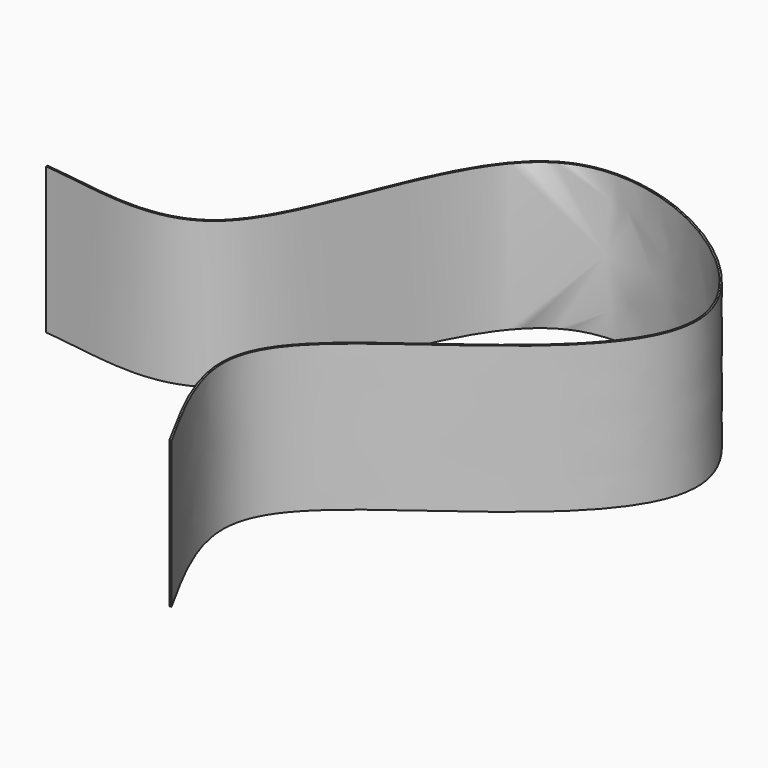
from build123d import *

# Parameters (mm, degrees)
F0_W     = 100
F0_H     = 70
F1_DEPTH = 16
F3_DEPTH = 25
F4_T     = -0.2
F5_DEPTH = 1


# Not quite as in the source:
# - a feature names something its author has since deleted; it is built from what else it names


with BuildPart() as f1:
    # F0 (on Top) → F1 (new body)
    with BuildSketch(Plane.XY):
        with Locations((0.9821429849, 33.5462264796)):
            Rectangle(F0_W, F0_H)
    extrude(amount=F1_DEPTH)

    # F2 (on face) → F3 (cut)
    with BuildSketch(Plane.XY.offset(16)):
        with BuildLine():
            Line((-49.0178570151, 68.5462264796), (-49.0178570151, 32.7192223562))
            add(Edge.make_bspline(
                [(-49.0178570151, 32.7192223562), (-43.4292364383, 32.2301652848), (-25.9811441186, 26.5813131518), (-21.7780426464, 74.7917895904), (26.8126262734, 45.2777093392), (-8.5734588785, 24.5947279779), (-17.4776549017, 13.6217093611), (-10.3822594237, 2.3846505635), (-8.3802593872, -1.4537735204)],
                knots=[0, 0, 0, 0, 0.1488243606, 0.3481063954, 0.5419458019, 0.7332399063, 0.8617053586, 1, 1, 1, 1], degree=3))
            Line((-8.3802593872, -1.4537735204), (50.9821429849, -1.4537735204))
            Line((50.9821429849, -1.4537735204), (50.9821429849, 68.5462264796))
            Line((50.9821429849, 68.5462264796), (-49.0178570151, 68.5462264796))
        make_face()
    extrude(amount=-F3_DEPTH, mode=Mode.SUBTRACT)

    # F4
    f4_openings = [f1.faces().sort_by_distance(p)[0] for p in [
        (-20.309609, 28.197223, 16),
        (-20.315883, 28.187702, 0),
        (-49.017857, 15.632724, 8),
    ]]
    offset(amount=F4_T, openings=f4_openings, kind=Kind.INTERSECTION)

    # F5 (cut): a face of the model
    f5_faces = [f1.faces().sort_by_distance(p)[0] for p in [
        (-28.6990582012, -1.4537735204, 8),
    ]]
    extrude(f5_faces, amount=-F5_DEPTH, mode=Mode.SUBTRACT)


solid = f1.part
